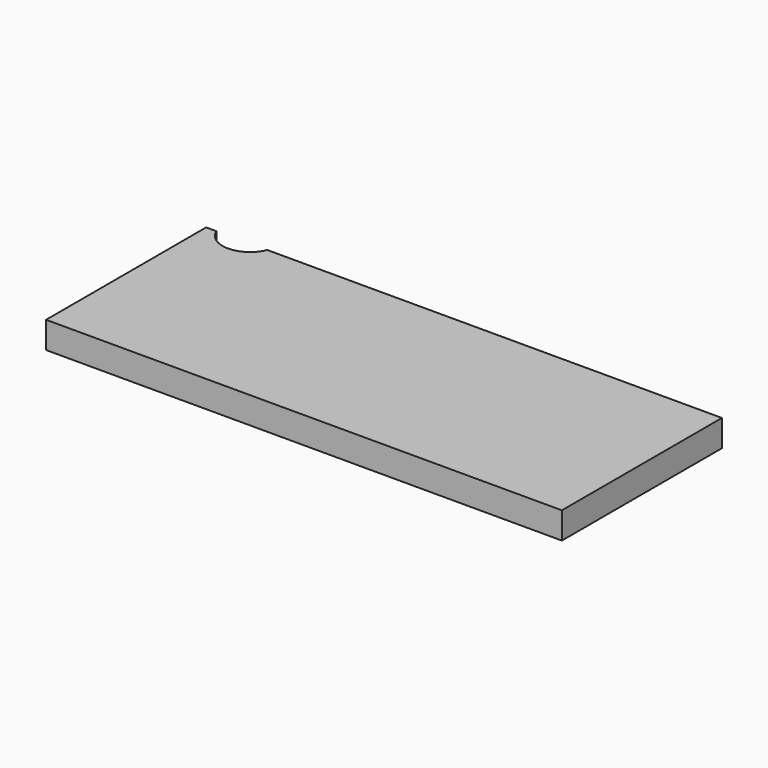
from build123d import *

# Parameters (mm, degrees)
F0_W     = 98.2365459204
F0_H     = 38.1
F1_DEPTH = 5.08
F3_DEPTH = 25.4


# Not quite as in the source:
# - a feature names something its author has since deleted; it is built from what else it names


with BuildPart() as f1:
    # F0 (on Top) → F1 (new body)
    with BuildSketch(Plane.XY):
        with Locations((0.2698786557, -21.017140013)):
            Rectangle(F0_W, F0_H)
    extrude(amount=F1_DEPTH)

    # F2 (on face) → F3 (cut)
    with BuildSketch(Plane.XY.offset(5.08)):
        with BuildLine():
            Line((-37.191967051, -1.967140013), (-46.9076386285, -1.967140013))
            ThreePointArc((-46.9076386285, -1.967140013), (-42.0498028398, -5.2410121524), (-37.191967051, -1.967140013))
        make_face()
        with BuildLine():
            ThreePointArc((-37.191967051, -1.967140013), (-36.9054766067, -1.0020558812), (-36.8087906874, 0))
            ThreePointArc((-36.8087906874, 0), (-43.051858721, 5.1443262331), (-46.9076386285, -1.967140013))
            Line((-46.9076386285, -1.967140013), (-37.191967051, -1.967140013))
        make_face()
    extrude(amount=-F3_DEPTH, mode=Mode.SUBTRACT)


solid = f1.part
